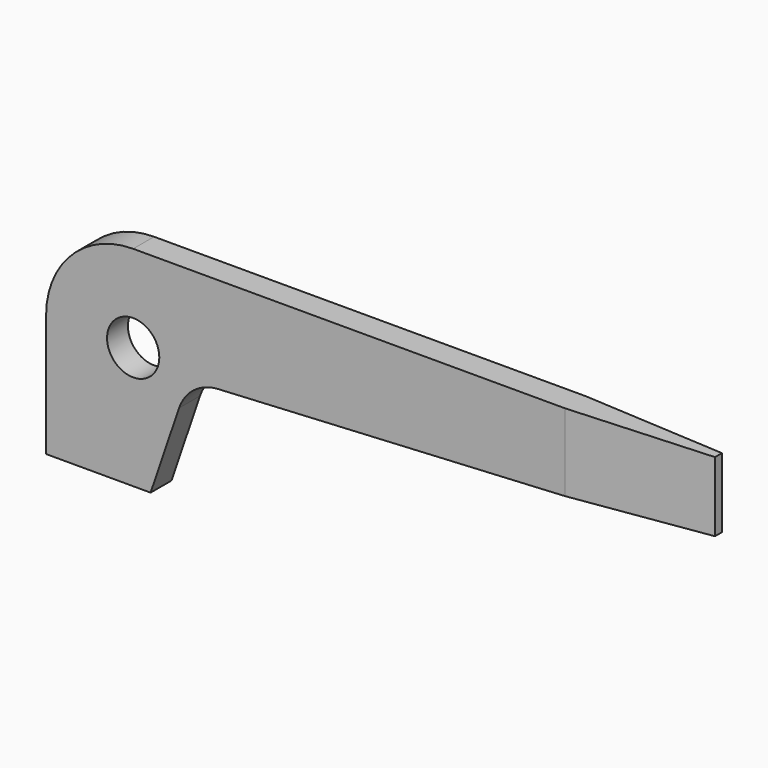
from build123d import *

# Parameters (mm, degrees)
F1_DEPTH = 2.38125
F2_R     = 2.38125
F3_DEPTH = 2.38225
F5_DEPTH = 25.4


# Not quite as in the source:
# - a length typed as a fraction of an inch, garbled in the dataset ("3 / 203.2 mm" for 3/8 in), is restored


with BuildPart() as f1:
    # F0 (on Front) → F1 (new body)
    with BuildSketch(Plane.XZ):
        with BuildLine():
            Line((60.325, 19.05), (7.9375, 19.05))
            ThreePointArc((7.9375, 19.05), (2.3248399243, 16.7251600757), (0, 11.1125))
            Line((0, 11.1125), (0, 0))
            Line((0, 0), (9.525, 0))
            Line((9.525, 0), (12.1173647876, 7.6271664624))
            ThreePointArc((12.1173647876, 7.6271664624), (13.4786145605, 9.5135918491), (15.6631963617, 10.3130942181))
            Line((15.6631963617, 10.3130942181), (60.325, 12.7))
            Line((60.325, 12.7), (60.325, 19.05))
        make_face()
    extrude(amount=F1_DEPTH)

    # F2 (on face) → F3 (cut, through all)
    with BuildSketch(Plane.XZ.offset(2.38125)):
        with Locations((7.9375, 11.1125)):
            Circle(F2_R)
    extrude(amount=-F3_DEPTH, mode=Mode.SUBTRACT)

    # F4 (on face) → F5 (cut)
    with BuildSketch(Plane.XY.offset(19.05)):
        Polygon((60.325, 0), (47.2817567568, 0), (60.325, -0.79375), align=None)
        Polygon((60.325, -2.38125), (60.325, -1.5875), (47.2817567568, -2.38125), align=None)
    extrude(amount=-F5_DEPTH, mode=Mode.SUBTRACT)


solid = f1.part
